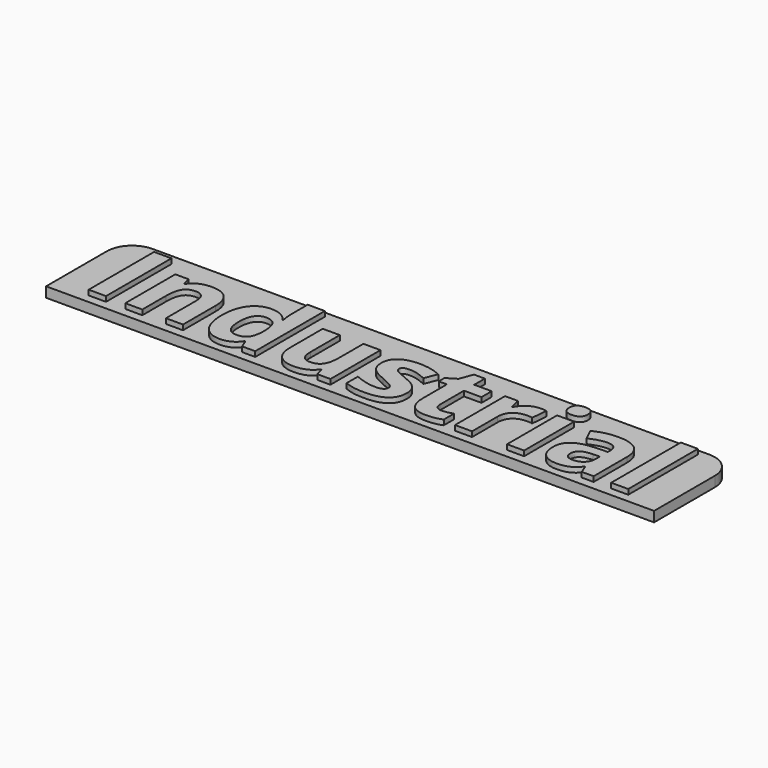
from build123d import *

# Parameters (mm, degrees)
F0_W         = 120
F0_H         = 20
F1_DEPTH     = 2
F2_TEXT_SIZE = 22.6126618058
F3_DEPTH     = 1
F4_R         = 5


# Not quite as in the source:
# - Text() gives the source's letters only with a copy of the font that has no kerning and outlines rounded to 1/6400 em; it was checked with that copy


with BuildPart() as f1:
    # F0 (on Top) → F1 (new body)
    with BuildSketch(Plane.XY):
        Rectangle(F0_W, F0_H)
    extrude(amount=F1_DEPTH)

    # F2 (on face) → F3 (join)
    with BuildSketch(Plane.XY.offset(2)):
        with Locations((-55, -8.2811165002)):
            Text('Industrial', F2_TEXT_SIZE, font='Open Sans', font_style=FontStyle.BOLD, text_align=(TextAlign.LEFT, TextAlign.BOTTOM))
    extrude(amount=F3_DEPTH)

    # F4
    f4_edges = [f1.edges().sort_by_distance(p)[0] for p in [
        (-60, 10, 1),
        (60, 10, 1),
    ]]
    fillet(f4_edges, radius=F4_R)


solid = f1.part
